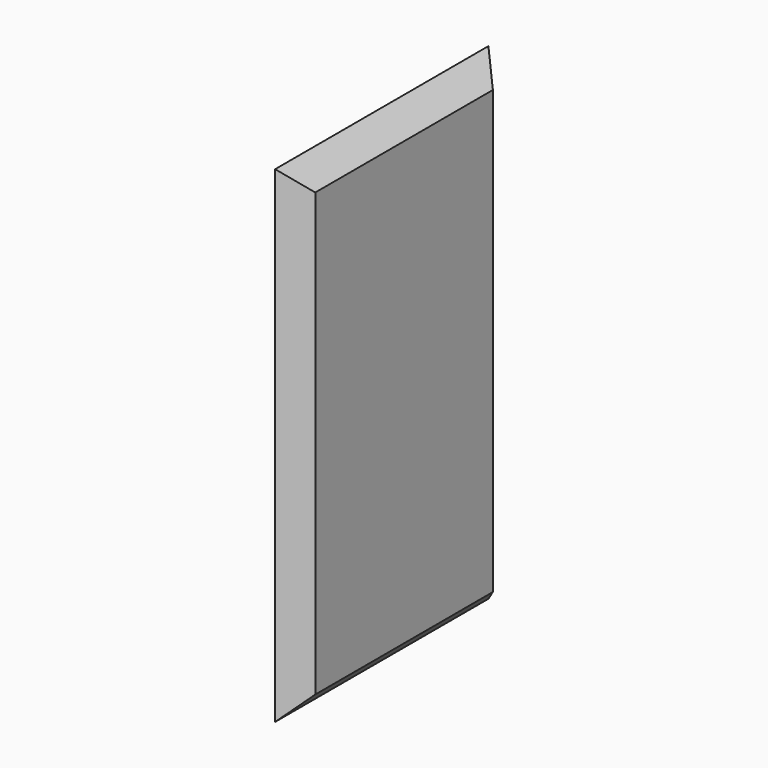
from build123d import *

# Parameters (mm, degrees)
F0_W     = 263
F0_H     = 480
F1_DEPTH = 22
F2_SIZE  = 21.99999


# Not quite as in the source:
# - a fillet or chamfer is up to 0.001 mm smaller than in the source, because OpenCascade refuses the exact size


with BuildPart() as f1:
    # F0 (on Right) → F1 (new body)
    with BuildSketch(Plane.YZ):
        Rectangle(F0_W, F0_H)
    extrude(amount=F1_DEPTH)

    # F2 (size 22 in the source; OpenCascade refuses exactly that, so slightly less here)
    f2_edges = [f1.edges().sort_by_distance(p)[0] for p in [
        (22, -131.5, 0),
        (22, 0, -240),
        (22, 131.5, 0),
        (22, 0, 240),
    ]]
    chamfer(f2_edges, length=F2_SIZE)


solid = f1.part
